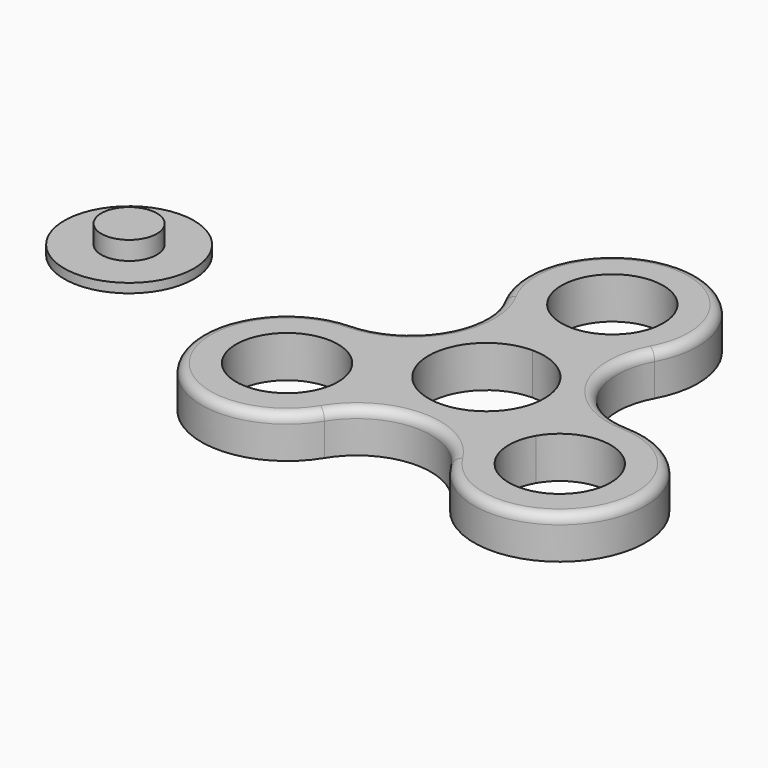
from build123d import *

# Parameters (mm, degrees)
F1_DEPTH = 4.5
F2_R     = 3
F3_DEPTH = 2
F2_R_2   = 7
F4_DEPTH = 1
F5_R     = 1


with BuildPart() as f1:
    # F0 (on Top) → F1 (new body)
    with BuildSketch(Plane.XY):
        with BuildLine():
            ThreePointArc((14.9497868783, 0.7472055075), (8.2182150114, 4.7447886491), (8.1219923905, 12.573292464))
            ThreePointArc((8.1219923905, 12.573292464), (0, 26.25), (-8.1219923905, 12.573292464))
            ThreePointArc((-8.1219923905, 12.573292464), (-8.2182150114, 4.7447886491), (-14.9497868783, 0.7472055075))
            ThreePointArc((-14.9497868783, 0.7472055075), (-22.7331668493, -13.125), (-6.8277944878, -13.3204979715))
            ThreePointArc((-6.8277944878, -13.3204979715), (0, -9.4895772982), (6.8277944878, -13.3204979715))
            ThreePointArc((6.8277944878, -13.3204979715), (22.7331668493, -13.125), (14.9497868783, 0.7472055075))
        make_face()
        with BuildLine():
            ThreePointArc((-9.2224318643, -8.5), (-20.0350239089, -9.9235047481), (-9.9592921435, -5.75))
            ThreePointArc((-9.9592921435, -5.75), (-9.4098398197, -7.0764952519), (-9.2224318643, -8.5))
        make_face(mode=Mode.SUBTRACT)
        with BuildLine():
            ThreePointArc((0, 6.25), (4.4194173824, 4.4194173824), (6.25, 0))
            ThreePointArc((6.25, 0), (6.0370364143, -1.6176190319), (5.4126587737, -3.125))
            ThreePointArc((5.4126587737, -3.125), (0, -6.25), (-5.4126587737, -3.125))
            ThreePointArc((-5.4126587737, -3.125), (-5.4126587737, 3.125), (0, 6.25))
        make_face(mode=Mode.SUBTRACT)
        with BuildLine():
            ThreePointArc((20.2224318643, -8.5), (13.2989271163, -13.8125920446), (9.9592921435, -5.75))
            ThreePointArc((9.9592921435, -5.75), (16.1459366124, -3.1874079554), (20.2224318643, -8.5))
        make_face(mode=Mode.SUBTRACT)
        with BuildLine():
            ThreePointArc((5.5, 17), (3.8890872965, 13.1109127035), (0, 11.5))
            ThreePointArc((0, 11.5), (-3.8890872965, 20.8890872965), (5.5, 17))
        make_face(mode=Mode.SUBTRACT)
    extrude(amount=F1_DEPTH)

    # F5
    f5_edges = [f1.edges().sort_by_distance(p)[0] for p in [
        (0, -9.489577, 4.5),
        (-22.733167, -13.125, 4.5),
        (-8.218215, 4.744789, 4.5),
        (0, 26.25, 4.5),
        (8.218215, 4.744789, 4.5),
        (22.733167, -13.125, 4.5),
    ]]
    fillet(f5_edges, radius=F5_R)


with BuildPart() as f3:
    # F2 (on Top) → F3 (new body)
    with BuildSketch(Plane.XY):
        with Locations((-44.0415814519, 6.8307667971)):
            Circle(F2_R)
    extrude(amount=F3_DEPTH)

    # F2 (on Top) → F4 (join)
    with BuildSketch(Plane.XY):
        with Locations((-44.0415814519, 6.8307667971)):
            Circle(F2_R_2)
        with Locations((-44.0415814519, 6.8307667971)):
            Circle(F2_R, mode=Mode.SUBTRACT)
        with Locations((-44.0415814519, 6.8307667971)):
            Circle(F2_R)
    extrude(amount=-F4_DEPTH)


solid = Compound([f1.part, f3.part])
